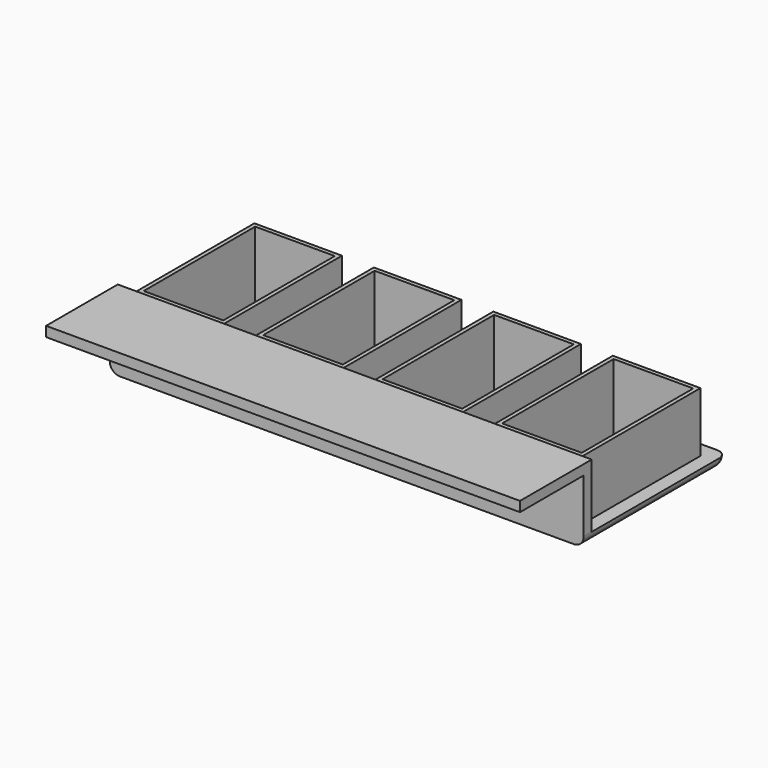
from build123d import *

# Parameters (mm, degrees)
F0_W     = 44
F0_H     = 74
F1_DEPTH = 5
F2_W     = 5
F2_H     = 27
F3_DEPTH = 238
F0_W_2   = 40
F0_H_2   = 70
F4_DEPTH = 35
F5_R     = 4.99999


# Not quite as in the source:
# - a fillet or chamfer is up to 0.001 mm smaller than in the source, because OpenCascade refuses the exact size


with BuildPart() as f1:
    # F0 (on Top) → F1 (new body)
    with BuildSketch(Plane.XY):
        Polygon((106.4276799491, 10), (-131.5723200509, 10), (-131.5723200509, -80), (-129.5723200509, -80), (106.4276799491, -80), align=None)
        with Locations((-102.5723200509, -35)):
            Rectangle(F0_W, F0_H, mode=Mode.SUBTRACT)
        with Locations((-42.5723200509, -35)):
            Rectangle(F0_W, F0_H, mode=Mode.SUBTRACT)
        with Locations((17.4276799491, -35)):
            Rectangle(F0_W, F0_H, mode=Mode.SUBTRACT)
        with Locations((77.4276799491, -35)):
            Rectangle(F0_W, F0_H, mode=Mode.SUBTRACT)
    extrude(amount=F1_DEPTH)

    # F2 (on face) → F3 (join)
    with BuildSketch(Plane(origin=(-131.5723200509, 0, 0), x_dir=(0, -1, 0), z_dir=(-1, 0, 0))):
        Polygon((120, 32), (120, 37), (75, 37), (75, 32), (80, 32), align=None)
        with Locations((77.5, 18.5)):
            Rectangle(F2_W, F2_H)
    extrude(amount=-F3_DEPTH)

    # F0 (on Top) → F4 (join)
    with BuildSketch(Plane.XY):
        with Locations((-102.5723200509, -35)):
            Rectangle(F0_W, F0_H)
        with Locations((-102.5723200509, -35)):
            Rectangle(F0_W_2, F0_H_2, mode=Mode.SUBTRACT)
        with Locations((-42.5723200509, -35)):
            Rectangle(F0_W, F0_H)
        with Locations((-42.5723200509, -35)):
            Rectangle(F0_W_2, F0_H_2, mode=Mode.SUBTRACT)
        with Locations((17.4276799491, -35)):
            Rectangle(F0_W, F0_H)
        with Locations((17.4276799491, -35)):
            Rectangle(F0_W_2, F0_H_2, mode=Mode.SUBTRACT)
        with Locations((77.4276799491, -35)):
            Rectangle(F0_W, F0_H)
        with Locations((77.4276799491, -35)):
            Rectangle(F0_W_2, F0_H_2, mode=Mode.SUBTRACT)
    extrude(amount=F4_DEPTH)

    # F5 (radius 5 in the source; OpenCascade refuses exactly that, so slightly less here)
    f5_edges = [f1.edges().sort_by_distance(p)[0] for p in [
        (-12.57232, 10, 0),
        (-131.57232, -35, 0),
        (106.42768, -35, 0),
        (106.42768, 10, 2.5),
        (-131.57232, 10, 2.5),
    ]]
    fillet(f5_edges, radius=F5_R)


solid = f1.part
